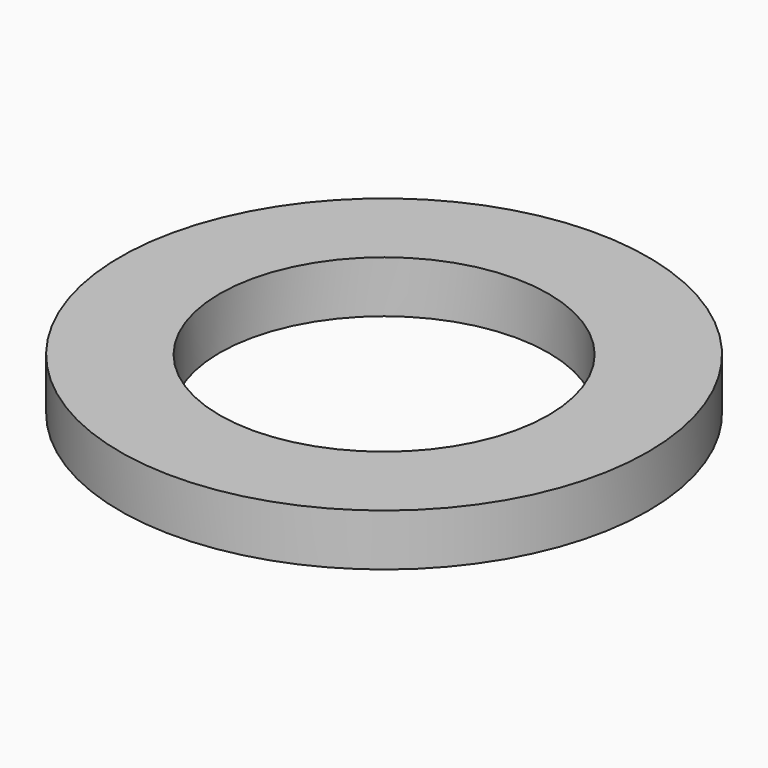
from build123d import *

# Parameters (mm, degrees)
F0_R     = 15.25
F0_R_2   = 9.5
F1_DEPTH = 3


# Not quite as in the source:
# - a feature names something its author has since deleted; it is built from what else it names


with BuildPart() as f1:
    # F0 (on Top) → F1 (new body)
    with BuildSketch(Plane.XY):
        with Locations((-39.1464792192, 0)):
            Circle(F0_R)
        with Locations((-39.1464792192, 0)):
            Circle(F0_R_2, mode=Mode.SUBTRACT)
    extrude(amount=F1_DEPTH)


solid = f1.part
